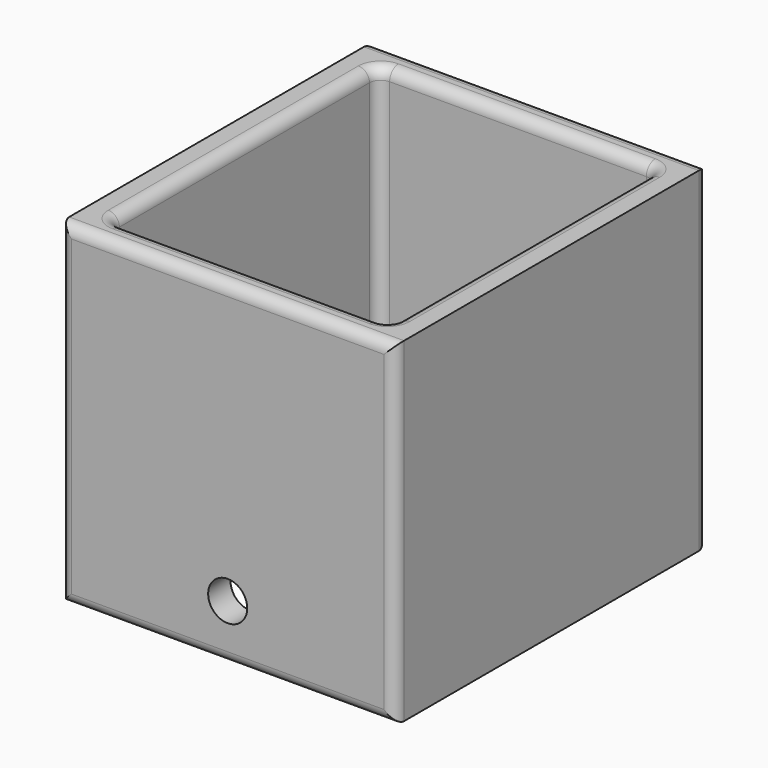
from build123d import *

# Parameters (mm, degrees)
F0_W     = 60
F0_H     = 70
F0_W_2   = 50
F0_H_2   = 60
F1_DEPTH = 60
F2_F1_R  = 2
F2_F2_R  = 2
F4_R     = 3.5
F5_DEPTH = 70


with BuildPart() as f1:
    # F0 (on Top) → F1 (new body)
    with BuildSketch(Plane.XY):
        Rectangle(F0_W, F0_H)
        Rectangle(F0_W_2, F0_H_2, mode=Mode.SUBTRACT)
    extrude(amount=F1_DEPTH)

    # F2: fillet of radius 2 on 16 edges, made by hand

    # F2_f1
    f2_f1_edges = [f1.edges().sort_by_distance(p)[0] for p in [
        (-25, -30, 30),
        (25, -30, 30),
        (25, 30, 30),
        (-25, 30, 30),
    ]]
    fillet(f2_f1_edges, radius=F2_F1_R)

    # F2_f2
    f2_f2_edges = [f1.edges().sort_by_distance(p)[0] for p in [
        (-30, 35, 30),
        (0, 35, 60),
        (30, 35, 30),
        (0, 35, 0),
        (30, -35, 30),
        (0, -35, 60),
        (-30, -35, 30),
        (0, -35, 0),
        (0, -30, 60),
        (0, -30, 0),
        (0, 30, 60),
        (0, 30, 0),
        (-24.4142135624, 29.4142135624, 0),
        (24.4142135624, 29.4142135624, 0),
        (-24.4142135624, 29.4142135624, 60),
        (24.4142135624, 29.4142135624, 60),
        (24.4142135624, -29.4142135624, 0),
        (-24.4142135624, -29.4142135624, 0),
        (24.4142135624, -29.4142135624, 60),
        (-24.4142135624, -29.4142135624, 60),
    ]]
    fillet(f2_f2_edges, radius=F2_F2_R)

    # F4 (on face) → F5 (cut)
    with BuildSketch(Plane(origin=(0, 35, 0), x_dir=(-1, 0, 0), z_dir=(0, 1, 0))):
        with Locations((0, 10)):
            Circle(F4_R)
    extrude(amount=-F5_DEPTH, mode=Mode.SUBTRACT)


solid = f1.part
